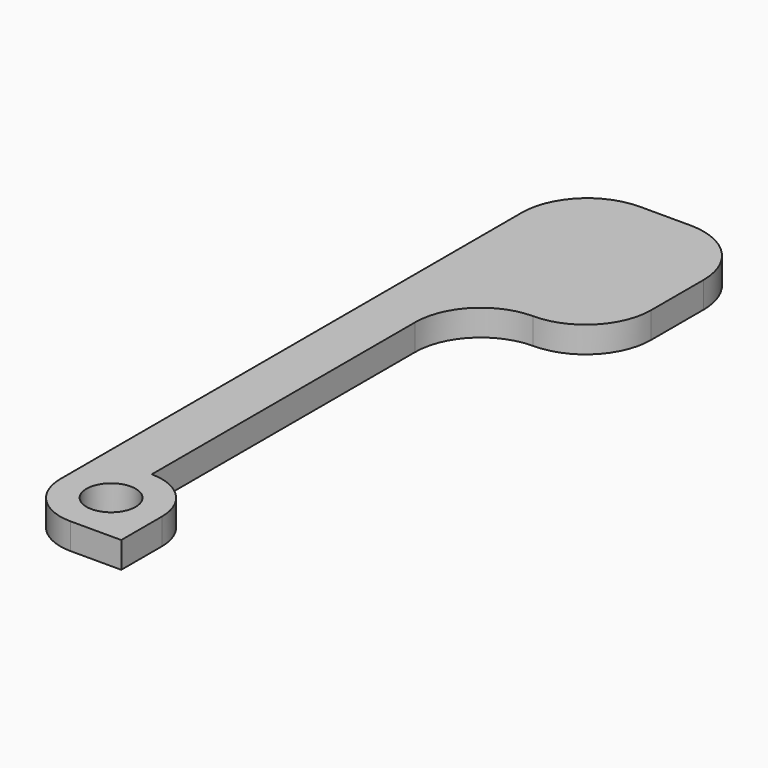
from build123d import *

# Parameters (mm, degrees)
F0_R     = 1.875
F1_DEPTH = 2
F2_R     = 4.99999


# Not quite as in the source:
# - a fillet or chamfer is up to 0.001 mm smaller than in the source, because OpenCascade refuses the exact size


with BuildPart() as f1:
    # F0 (on Top) → F1 (new body)
    with BuildSketch(Plane.XY):
        with BuildLine():
            ThreePointArc((0, 3.876953125), (-2.741419845, 2.741419845), (-3.876953125, 0))
            ThreePointArc((-3.876953125, 0), (-2.741419845, -2.741419845), (0, -3.876953125))
            ThreePointArc((0, -3.876953125), (2.741419845, -2.741419845), (3.876953125, 0))
            ThreePointArc((3.876953125, 0), (2.741419845, 2.741419845), (0, 3.876953125))
        make_face()
        Circle(F0_R, mode=Mode.SUBTRACT)
        with BuildLine():
            Line((-3.876953125, 49), (-3.876953125, 0))
            ThreePointArc((-3.876953125, 0), (-2.741419845, 2.741419845), (0, 3.876953125))
            Line((0, 3.876953125), (0, 34))
            Line((0, 34), (10, 34))
            Line((10, 34), (10, 49))
            Line((10, 49), (-3.876953125, 49))
        make_face()
        with BuildLine():
            ThreePointArc((3.876953125, 0), (2.741419845, -2.741419845), (0, -3.876953125))
            Line((0, -3.876953125), (3.876953125, -3.876953125))
            Line((3.876953125, -3.876953125), (3.876953125, 0))
        make_face()
    extrude(amount=F1_DEPTH)

    # F2 (radius 5 in the source; OpenCascade refuses exactly that, so slightly less here)
    f2_edges = [f1.edges().sort_by_distance(p)[0] for p in [
        (0, 34, 1),
        (10, 34, 1),
        (10, 49, 1),
        (-3.876953, 49, 1),
    ]]
    fillet(f2_edges, radius=F2_R)


solid = f1.part
